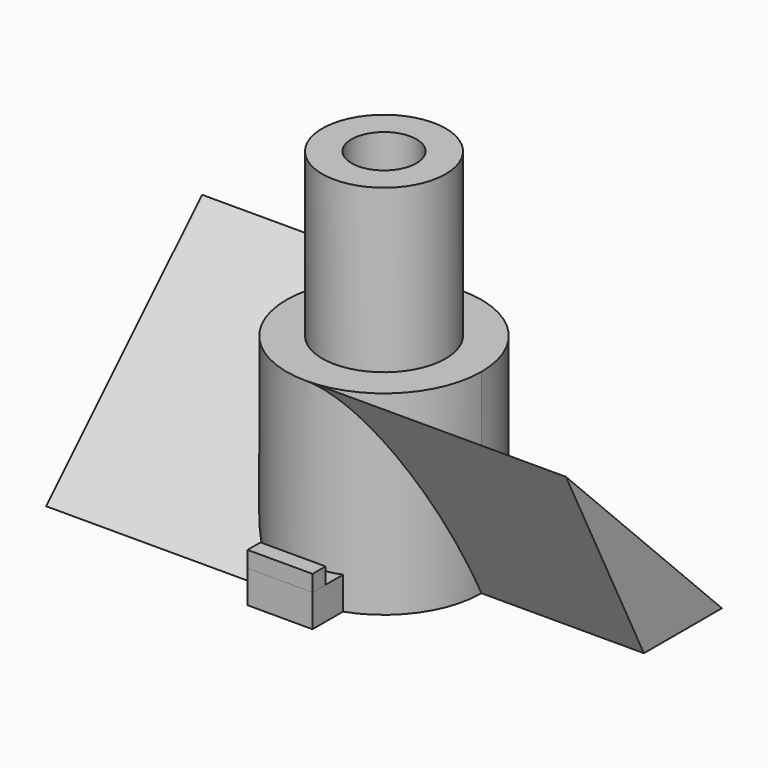
from build123d import *
from build123d import SkipClean  # not in build123d's __all__

# Parameters (mm, degrees)
F0_R      = 7.62
F1_DEPTH  = 15.24
F3_DEPTH  = 20.32
F5_COUNT  = 2
F6_W      = 5.0799995622
F6_H      = 2.54
F7_DEPTH  = 10.16
F8_W      = 5.0799995622
F8_H      = 1.27
F9_DEPTH  = 1.27
F10_R     = 2.54
F11_DEPTH = 15.241
F12_R     = 4.826
F12_R_2   = 2.54
F13_DEPTH = 12.7


with BuildPart() as f1:
    # F0 (on Top) → F1 (new body)
    with BuildSketch(Plane.XY):
        Circle(F0_R)
    extrude(amount=F1_DEPTH)



with BuildPart() as f3:
    # F2 (on Right) → F3 (new body)
    with BuildSketch(Plane.YZ):
        Polygon((-7.62, 15.24), (0, 0), (7.62, 0), align=None)
    extrude(amount=F3_DEPTH)


with BuildPart() as f1_1:
    add(f1.part, clean=False)

    with SkipClean():  # cleaning this boolean's faces spoils the solid; the shape is the same uncleaned
        add(f3.part)  # F5 merges F3
    # F5: F3 ×2 about axis
    f5_axis = Axis((0, 0, 17.5851359963), (0, 0, 1))
    with SkipClean():  # cleaning this boolean's faces spoils the solid; the shape is the same uncleaned
        for i in range(1, F5_COUNT):
            add(f3.part.rotate(f5_axis, i * 360 / F5_COUNT), clean=False)

    # F6 (on Front) → F7 (join)
    with BuildSketch(Plane.XZ):
        with Locations((0, 1.27)):
            Rectangle(F6_W, F6_H)
    with SkipClean():  # cleaning this boolean's faces spoils the solid; the shape is the same uncleaned
        extrude(amount=F7_DEPTH)

    # F8 (on face) → F9 (join)
    with BuildSketch(Plane.XY.offset(2.54)):
        with Locations((0, -9.525)):
            Rectangle(F8_W, F8_H)
    with SkipClean():  # cleaning this boolean's faces spoils the solid; the shape is the same uncleaned
        extrude(amount=F9_DEPTH)

    # F10 (on face) → F11 (cut, through all)
    with BuildSketch(Plane.XY.offset(15.24)):
        Circle(F10_R)
    with SkipClean():  # cleaning this boolean's faces spoils the solid; the shape is the same uncleaned
        extrude(amount=-F11_DEPTH, mode=Mode.SUBTRACT)

    # F12 (on face) → F13 (join)
    with BuildSketch(Plane.XY.offset(15.24)):
        Circle(F12_R)
        Circle(F12_R_2, mode=Mode.SUBTRACT)
    with SkipClean():  # cleaning this boolean's faces spoils the solid; the shape is the same uncleaned
        extrude(amount=F13_DEPTH)


solid = f1_1.part
